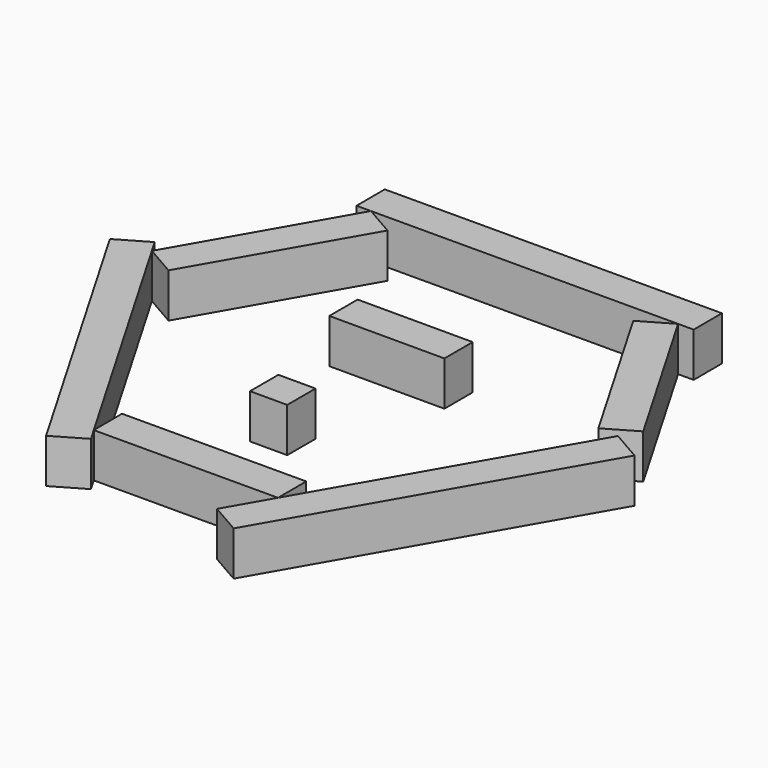
from build123d import *

# Parameters (mm, degrees)
F1_DEPTH = 25
F2_DEPTH = 25
F0_W     = 65
F0_H     = 20
F3_DEPTH = 25
F0_W_2   = 21


# Not quite as in the source:
# - a feature names something its author has since deleted; it is built from what else it names


with BuildPart() as f1:
    # F0 (on Top) → F1 (new body)
    with BuildSketch(Plane.XY):
        Polygon((-69.4846216079, 99.7250617094), (-86.8309071217, 109.6802803847), (-138.504703636, 19.6422352991), (-121.1584181221, 9.6870166238), align=None)
    extrude(amount=F1_DEPTH)


with BuildPart() as f1b:
    # F0 (on Top) → F1, piece 2 (new body)
    with BuildSketch(Plane.XY):
        Polygon((94.9996829561, 130.1501124276), (0, 129.9046776291), (-94.9996829561, 129.6592428305), (-94.9480124722, 109.6593095766), (-86.8309071217, 109.6802803847), (-63.7681405371, 109.739863799), (86.2630265741, 110.1274742428), (95.05135344, 110.1501791737), align=None)
    extrude(amount=F1_DEPTH)


with BuildPart() as f1c:
    # F0 (on Top) → F1, piece 3 (new body)
    with BuildSketch(Plane.XY):
        Polygon((138.4013626682, 20.3576312087), (86.2630265741, 110.1274742428), (68.9684115442, 100.0827596642), (121.1067476382, 10.3129166301), align=None)
    extrude(amount=F1_DEPTH)


with BuildPart() as f1d:
    # F0 (on Top) → F1, piece 4 (new body)
    with BuildSketch(Plane.XY):
        Polygon((-51.6221260304, -110.0379783395), (-51.5704555465, -130.0379115934), (52.2416770618, -129.769709542), (52.1900065779, -109.769776288), align=None)
    extrude(amount=F1_DEPTH)


with BuildPart() as f1e:
    # F0 (on Top) → F1, piece 5 (new body)
    with BuildSketch(Plane.XY):
        Polygon((-51.5704555465, -130.0379115934), (-138.504703636, 19.6422352991), (-142.7499738398, 26.951583245), (-160.0445888697, 16.9068686664), (-112.3321946212, -65.2425527258), (-64.6198003726, -147.391974118), (-47.3251853427, -137.3472595393), align=None)
    extrude(amount=F1_DEPTH)


with BuildPart() as f2:
    # F0 (on Top) → F2 (new body)
    with BuildSketch(Plane.XY):
        Polygon((132.4313069212, 9.9552186753), (52.2416770618, -129.769709542), (37.8567295061, -154.8344937062), (55.2030150199, -164.7897123814), (102.4903037275, -82.3948561907), (149.7775924351, 0), align=None)
    extrude(amount=F2_DEPTH)


with BuildPart() as f3:
    # F0 (on Top) → F3 (new body)
    with BuildSketch(Plane.XY):
        with Locations((-6.0981351137, 29.9933182448)):
            Rectangle(F0_W, F0_H)
    extrude(amount=F3_DEPTH)


with BuildPart() as f3b:
    # F0 (on Top) → F3, piece 2 (new body)
    with BuildSketch(Plane.XY):
        with Locations((-10.5, -47.9548701644)):
            Rectangle(F0_W_2, F0_H)
    extrude(amount=F3_DEPTH)


solid = Compound([f1.part, f1b.part, f1c.part, f1d.part, f1e.part, f2.part, f3.part, f3b.part])
